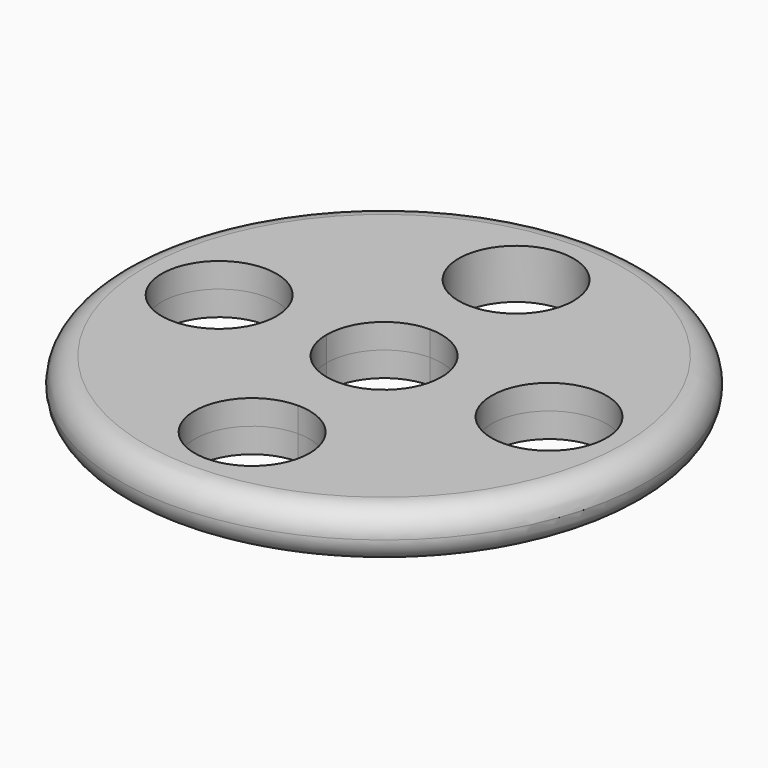
from build123d import *

# Parameters (mm, degrees)
F0_R     = 50.8
F0_R_2   = 11.049
F1_DEPTH = 4.7625
F2_R     = 4.76249


# Not quite as in the source:
# - a fillet or chamfer is up to 0.001 mm smaller than in the source, because OpenCascade refuses the exact size


with BuildPart() as f1:
    # F0 (on Top) → F1 (new body, symmetric)
    with BuildSketch(Plane.XY):
        Circle(F0_R)
        with BuildLine():
            ThreePointArc((11.049, -31.75), (-7.8128228253, -39.5628228253), (0, -20.701))
            ThreePointArc((0, -20.701), (7.8128228253, -23.9371771747), (11.049, -31.75))
        make_face(mode=Mode.SUBTRACT)
        with Locations((-31.75, 0)):
            Circle(F0_R_2, mode=Mode.SUBTRACT)
        with BuildLine():
            ThreePointArc((0, 11.049), (7.8128228253, 7.8128228253), (11.049, 0))
            ThreePointArc((11.049, 0), (7.8128228253, -7.8128228253), (0, -11.049))
            ThreePointArc((0, -11.049), (-7.8128228253, -7.8128228253), (-11.049, 0))
            ThreePointArc((-11.049, 0), (-7.8128228253, 7.8128228253), (0, 11.049))
        make_face(mode=Mode.SUBTRACT)
        with BuildLine():
            ThreePointArc((42.799, 0), (31.75, -11.049), (20.701, 0))
            ThreePointArc((20.701, 0), (31.75, 11.049), (42.799, 0))
        make_face(mode=Mode.SUBTRACT)
        with BuildLine():
            ThreePointArc((11.049, 31.75), (7.8128228253, 23.9371771747), (0, 20.701))
            ThreePointArc((0, 20.701), (-7.8128228253, 39.5628228253), (11.049, 31.75))
        make_face(mode=Mode.SUBTRACT)
    extrude(amount=F1_DEPTH, both=True)

    # F2 (radius 4.7625 in the source; OpenCascade refuses exactly that, so slightly less here)
    f2_edges = [f1.edges().sort_by_distance(p)[0] for p in [
        (-50.8, 0, -4.7625),
        (50.8, 0, 0),
        (-50.8, 0, 4.7625),
    ]]
    fillet(f2_edges, radius=F2_R)


solid = f1.part
